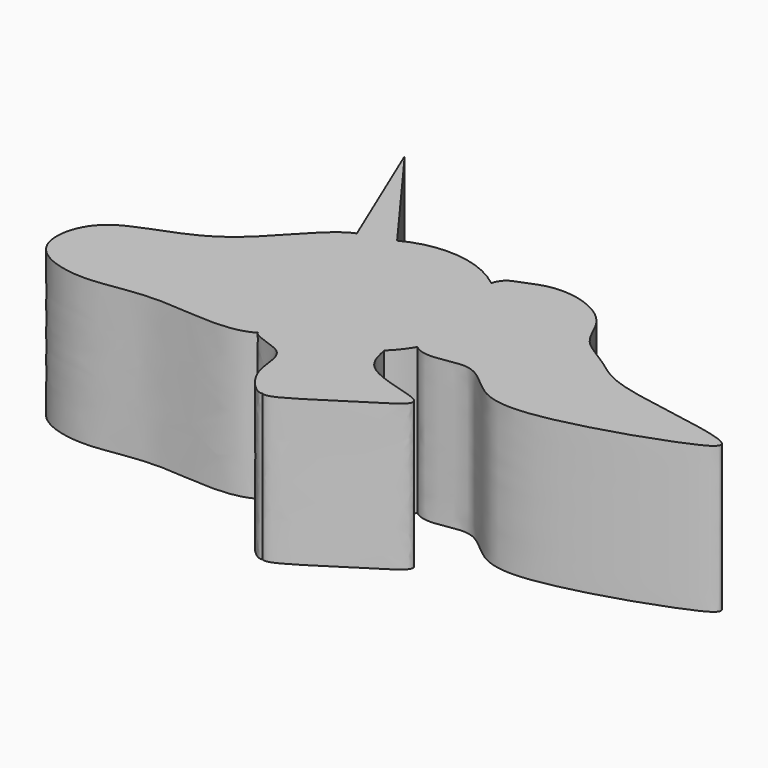
from build123d import *

# Parameters (mm, degrees)
F1_DEPTH = 25.4


with BuildPart() as f1:
    # F0 (on Top) → F1 (new body)
    with BuildSketch(Plane.XY):
        with BuildLine():
            ThreePointArc((15.6247597688, -17.5122784292), (16.158858904, -15.1511123847), (16.3382044071, -12.7369454131))
            ThreePointArc((16.3382044071, -12.7369454131), (14.732957367, -5.6745881247), (10.2326509171, 0))
            add(Edge.make_bspline(
                [(11.0694508842, -15.1028212661), (9.5993425881, -9.8895547332), (9.3093062782, -2.986619819), (10.2326509171, 0)],
                knots=[0.9266033138, 0.9266033138, 0.9266033138, 0.9266033138, 1, 1, 1, 1], degree=3))
            ThreePointArc((11.0694508842, -15.1028212661), (13.2014186834, -16.5829843604), (15.6247597688, -17.5122784292))
        make_face()
        with BuildLine():
            ThreePointArc((10.2326509171, 0), (14.732957367, -5.6745881247), (16.3382044071, -12.7369454131))
            ThreePointArc((16.3382044071, -12.7369454131), (16.158858904, -15.1511123847), (15.6247597688, -17.5122784292))
            ThreePointArc((15.6247597688, -17.5122784292), (24.9039357291, -15.5507675945), (29.064724865, -7.0279473439))
            ThreePointArc((29.064724865, -7.0279473439), (22.2178667073, 3.0289081499), (10.3511869131, 0.3453061453))
            add(Edge.make_bspline(
                [(10.2326509171, 0), (10.2701911189, 0.1214262863), (10.3097370055, 0.2363790128), (10.3511869131, 0.3453061453)],
                knots=[0, 0, 0, 0, 0.0029840715, 0.0029840715, 0.0029840715, 0.0029840715], degree=3))
        make_face()
        with BuildLine():
            add(Edge.make_bspline(
                [(11.0694508842, -15.1028212661), (9.5993425881, -9.8895547332), (9.3093062782, -2.986619819), (10.2326509171, 0)],
                knots=[0.9266033138, 0.9266033138, 0.9266033138, 0.9266033138, 1, 1, 1, 1], degree=3))
            ThreePointArc((10.2326509171, 0), (10.1764969932, 0.0449101719), (10.1201459651, 0.0895727775))
            ThreePointArc((10.1201459651, 0.0895727775), (7.4671185374, -7.7020590055), (11.0694508842, -15.1028212661))
        make_face()
        with BuildLine():
            ThreePointArc((29.064724865, -7.0279473439), (24.9039357291, -15.5507675945), (15.6247597688, -17.5122784292))
            ThreePointArc((15.6247597688, -17.5122784292), (14.97657106, -19.2668185001), (14.1320946898, -20.9357759959))
            add(Edge.make_bspline(
                [(10.3511869131, 0.3453061453), (10.9660918821, 1.9612285661), (13.1810710321, 2.5821615076), (17.4062250817, 4.5972614145), (23.5541211341, 4.0157306024), (29.1807841604, 0.4734658783), (30.6152690832, -5.6031749227), (37.2457146084, -8.7606918958), (41.6262591245, -13.5919512406), (69.4069767494, -16.0194865708), (58.4173073455, -21.3590816503), (43.2741615609, -26.3017495114), (29.7906561882, -27.9538614081), (23.9099000961, -18.8038777974), (16.6936052342, -23.0245011534), (14.1320946898, -20.9357759959)],
                knots=[0.0029840715, 0.0029840715, 0.0029840715, 0.0029840715, 0.0472524544, 0.0978197845, 0.156226181, 0.2156699733, 0.2729250454, 0.3328538195, 0.399296056, 0.5093923331, 0.5642444856, 0.6651313762, 0.7494833831, 0.8187715875, 0.8901220386, 0.8901220386, 0.8901220386, 0.8901220386], degree=3))
            ThreePointArc((10.3511869131, 0.3453061453), (22.2178667073, 3.0289081499), (29.064724865, -7.0279473439))
        make_face()
        with BuildLine():
            ThreePointArc((14.1320946898, -20.9357759959), (14.97657106, -19.2668185001), (15.6247597688, -17.5122784292))
            ThreePointArc((15.6247597688, -17.5122784292), (13.2014186834, -16.5829843604), (11.0694508842, -15.1028212661))
            add(Edge.make_bspline(
                [(14.1320946898, -20.9357759959), (12.8224019033, -19.8678169833), (11.8001572435, -17.6940364971), (11.0694508842, -15.1028212661)],
                knots=[0.8901220386, 0.8901220386, 0.8901220386, 0.8901220386, 0.9266033138, 0.9266033138, 0.9266033138, 0.9266033138], degree=3))
        make_face()
        with BuildLine():
            ThreePointArc((11.0694508842, -15.1028212661), (7.4671185374, -7.7020590055), (10.1201459651, 0.0895727775))
            ThreePointArc((10.1201459651, 0.0895727775), (1.5397794917, 3.5285395894), (-7.5334858124, 1.7607618112))
            ThreePointArc((-7.5334858124, 1.7607618112), (-8.9265880443, 0.947094529), (-10.2326509171, 0))
            add(Edge.make_bspline(
                [(-3.0699548582, -28.7841352111), (0.8240097012, -21.7530635718), (-4.4613062913, -2.497334585), (-10.2326509171, 0)],
                knots=[0.8075795969, 0.8075795969, 0.8075795969, 0.8075795969, 1, 1, 1, 1], degree=3))
            add(Edge.make_bspline(
                [(-1.0373402516, -29.0421853208), (-1.7263886536, -28.7488598338), (-2.411144298, -28.652496149), (-3.0699548582, -28.7841352111)],
                knots=[0.8274826523, 0.8274826523, 0.8274826523, 0.8274826523, 0.8828352089, 0.8828352089, 0.8828352089, 0.8828352089], degree=3))
            ThreePointArc((-1.0373402516, -29.0421853208), (0.2330522052, -29.0734875783), (1.5020347762, -29.0059593591))
            add(Edge.make_bspline(
                [(1.9966859836, -25.2967402339), (1.3467949947, -26.4147374297), (1.2639465735, -27.7023037912), (1.5020347762, -29.0059593591)],
                knots=[0, 0, 0, 0, 0.0539789023, 0.0539789023, 0.0539789023, 0.0539789023], degree=3))
            add(Edge.make_bspline(
                [(11.2626201962, -24.5729206396), (11.0063895855, -23.5189771031), (9.9645541492, -20.328136721), (3.5168312901, -22.6816582912), (1.9966859836, -25.2967402339)],
                knots=[0.8238879416, 0.8238879416, 0.8238879416, 0.8238879416, 0.873739171, 1, 1, 1, 1], degree=3))
            ThreePointArc((11.2626201962, -24.5729206396), (12.8269283667, -22.8565714892), (14.1320946898, -20.9357759959))
            add(Edge.make_bspline(
                [(14.1320946898, -20.9357759959), (12.8224019033, -19.8678169833), (11.8001572435, -17.6940364971), (11.0694508842, -15.1028212661)],
                knots=[0.8901220386, 0.8901220386, 0.8901220386, 0.8901220386, 0.9266033138, 0.9266033138, 0.9266033138, 0.9266033138], degree=3))
        make_face()
        with BuildLine():
            ThreePointArc((-10.2326509171, 0), (-8.9265880443, 0.947094529), (-7.5334858124, 1.7607618112))
            Line((-7.5334858124, 1.7607618112), (-22.2487710416, 21.8024943024))
            Line((-22.2487710416, 21.8024943024), (-13.127635327, 0))
            add(Edge.make_bspline(
                [(-10.2326509171, 0), (-11.1825010918, 0.4110123109), (-12.1455161813, 0.368094916), (-13.127635327, 0)],
                knots=[0, 0, 0, 0, 0.0316686258, 0.0316686258, 0.0316686258, 0.0316686258], degree=3))
        make_face()
        with BuildLine():
            add(Edge.make_bspline(
                [(6.2752948143, -44.7073355317), (7.4566317865, -45.6619770197), (16.6946003339, -38.7648248858), (28.6623877442, -32.6401294165), (12.4889474561, -31.4488202018), (11.6144968935, -26.0202815526), (11.2626201962, -24.5729206396)],
                knots=[0.3326677956, 0.3326677956, 0.3326677956, 0.3326677956, 0.483522904, 0.6092698166, 0.7554281822, 0.8238879416, 0.8238879416, 0.8238879416, 0.8238879416], degree=3))
            ThreePointArc((11.2626201962, -24.5729206396), (6.756260964, -27.6127600473), (1.5020347762, -29.0059593591))
            add(Edge.make_bspline(
                [(1.5020347762, -29.0059593591), (1.7582976885, -30.409130826), (2.3863654431, -31.8309416267), (3.0793600463, -33.0800123041)],
                knots=[0.0539789023, 0.0539789023, 0.0539789023, 0.0539789023, 0.1120783401, 0.1120783401, 0.1120783401, 0.1120783401], degree=3))
            add(Edge.make_bspline(
                [(3.7081294957, -34.1456867388), (3.5040593333, -33.7751099484), (3.2941622239, -33.4194445981), (3.0793600283, -33.0800122747)],
                knots=[0.6943378528, 0.6943378528, 0.6943378528, 0.6943378528, 0.7136660465, 0.7136660465, 0.7136660465, 0.7136660465], degree=3))
            add(Edge.make_bspline(
                [(3.7081294937, -34.1456867399), (4.9882228558, -36.1974885553), (6.3669138471, -37.6924416259), (6.2780647625, -40.2375798495), (6.2515850068, -40.5877476318)],
                knots=[0.1293935148, 0.1293935148, 0.1293935148, 0.1293935148, 0.2349709338, 0.2514569097, 0.2514569097, 0.2514569097, 0.2514569097], degree=3))
            add(Edge.make_bspline(
                [(6.2752948143, -44.7073355317), (6.8854909927, -44.3655439077), (6.7882111753, -42.687560365), (6.2515850082, -40.5877476332)],
                knots=[0.482945294, 0.482945294, 0.482945294, 0.482945294, 0.590468255, 0.590468255, 0.590468255, 0.590468255], degree=3))
        make_face()
        with BuildLine():
            ThreePointArc((1.5020347762, -29.0059593591), (6.756260964, -27.6127600473), (11.2626201962, -24.5729206396))
            add(Edge.make_bspline(
                [(11.2626201962, -24.5729206396), (11.0063895855, -23.5189771031), (9.9645541492, -20.328136721), (3.5168312901, -22.6816582912), (1.9966859836, -25.2967402339)],
                knots=[0.8238879416, 0.8238879416, 0.8238879416, 0.8238879416, 0.873739171, 1, 1, 1, 1], degree=3))
            add(Edge.make_bspline(
                [(1.9966859836, -25.2967402339), (1.3467949947, -26.4147374297), (1.2639465735, -27.7023037912), (1.5020347762, -29.0059593591)],
                knots=[0, 0, 0, 0, 0.0539789023, 0.0539789023, 0.0539789023, 0.0539789023], degree=3))
        make_face()
        with BuildLine():
            add(Edge.make_bspline(
                [(-3.0699548582, -28.7841352111), (0.8240097012, -21.7530635718), (-4.4613062913, -2.497334585), (-10.2326509171, 0)],
                knots=[0.8075795969, 0.8075795969, 0.8075795969, 0.8075795969, 1, 1, 1, 1], degree=3))
            ThreePointArc((-10.2326509171, 0), (-14.5067813584, -5.2209479499), (-16.3067587039, -11.7237604245))
            ThreePointArc((-16.3067587039, -11.7237604245), (-9.7227081214, -13.4309985411), (-6.8315372381, -19.5877440274))
            ThreePointArc((-6.8315372381, -19.5877440274), (-7.6120209178, -23.0344974741), (-9.8012018612, -25.808799349))
            ThreePointArc((-9.8012018612, -25.808799349), (-6.6052876316, -27.6804088185), (-3.0699548582, -28.7841352111))
        make_face()
        with BuildLine():
            ThreePointArc((-16.3067587039, -11.7237604245), (-14.5067813584, -5.2209479499), (-10.2326509171, 0))
            add(Edge.make_bspline(
                [(-10.2326509171, 0), (-11.1825010918, 0.4110123109), (-12.1455161813, 0.368094916), (-13.127635327, 0)],
                knots=[0, 0, 0, 0, 0.0316686258, 0.0316686258, 0.0316686258, 0.0316686258], degree=3))
            add(Edge.make_bspline(
                [(-13.127635327, 0), (-16.9885407298, -1.4470542155), (-26.1475214336, -15.710526233), (-43.4116839601, -16.662992314), (-45.950942929, -30.8867076179), (-33.5443465173, -34.5459712582), (-23.2656635988, -30.7793989739), (-9.4186082957, -33.630807497), (-5.3864327744, -31.188833942)],
                knots=[0.0316686258, 0.0316686258, 0.0316686258, 0.0316686258, 0.1561642831, 0.3060221782, 0.4153421079, 0.5268671977, 0.655086979, 0.7787124677, 0.7787124677, 0.7787124677, 0.7787124677], degree=3))
            add(Edge.make_bspline(
                [(-3.0699548582, -28.7841352111), (-4.4644595819, -29.062775696), (-5.7427193917, -30.362964597), (-5.3864327744, -31.188833942)],
                knots=[0.8828352089, 0.8828352089, 0.8828352089, 0.8828352089, 1, 1, 1, 1], degree=3))
            ThreePointArc((-3.0699548582, -28.7841352111), (-6.6052876316, -27.6804088185), (-9.8012018612, -25.808799349))
            ThreePointArc((-9.8012018612, -25.808799349), (-22.0961404136, -22.9426465286), (-16.3067587039, -11.7237604245))
        make_face()
        with BuildLine():
            add(Edge.make_bspline(
                [(1.5020347762, -29.0059593591), (1.7582976885, -30.409130826), (2.3863654431, -31.8309416267), (3.0793600463, -33.0800123041)],
                knots=[0.0539789023, 0.0539789023, 0.0539789023, 0.0539789023, 0.1120783401, 0.1120783401, 0.1120783401, 0.1120783401], degree=3))
            ThreePointArc((1.5020347762, -29.0059593591), (0.2330522052, -29.0734875783), (-1.0373402516, -29.0421853208))
            add(Edge.make_bspline(
                [(3.0793600463, -33.0800123041), (1.8144691163, -31.0812204976), (0.3794895238, -29.6453247849), (-1.0373402516, -29.0421853208)],
                knots=[0.7136660465, 0.7136660465, 0.7136660465, 0.7136660465, 0.8274826523, 0.8274826523, 0.8274826523, 0.8274826523], degree=3))
        make_face()
        with BuildLine():
            add(Edge.make_bspline(
                [(-5.3864327744, -31.188833942), (-4.908330002, -32.2970720971), (2.1683533748, -32.8226904652), (0.3871749857, -40.3054793101), (5.3800366063, -45.2088000896), (6.2752948143, -44.7073355317)],
                knots=[0, 0, 0, 0, 0.1572240121, 0.3251914161, 0.482945294, 0.482945294, 0.482945294, 0.482945294], degree=3))
            add(Edge.make_bspline(
                [(6.2515850082, -40.5877476332), (6.1211441743, -42.3126947019), (5.6393374171, -44.1934167006), (6.2752948143, -44.7073355317)],
                knots=[0.2514569097, 0.2514569097, 0.2514569097, 0.2514569097, 0.3326677956, 0.3326677956, 0.3326677956, 0.3326677956], degree=3))
            add(Edge.make_bspline(
                [(6.2515850082, -40.5877476332), (5.7331920658, -38.5592813245), (4.8048013486, -36.1371642314), (3.7081294957, -34.1456867388)],
                knots=[0.590468255, 0.590468255, 0.590468255, 0.590468255, 0.6943378528, 0.6943378528, 0.6943378528, 0.6943378528], degree=3))
            add(Edge.make_bspline(
                [(3.0793600463, -33.0800123041), (3.2858908332, -33.4522685219), (3.4981884, -33.8091819739), (3.7081294937, -34.1456867399)],
                knots=[0.1120783401, 0.1120783401, 0.1120783401, 0.1120783401, 0.1293935148, 0.1293935148, 0.1293935148, 0.1293935148], degree=3))
            add(Edge.make_bspline(
                [(3.0793600463, -33.0800123041), (1.8144691163, -31.0812204976), (0.3794895238, -29.6453247849), (-1.0373402516, -29.0421853208)],
                knots=[0.7136660465, 0.7136660465, 0.7136660465, 0.7136660465, 0.8274826523, 0.8274826523, 0.8274826523, 0.8274826523], degree=3))
            ThreePointArc((-1.0373402516, -29.0421853208), (-2.0576967086, -28.9450547261), (-3.0699548582, -28.7841352111))
            add(Edge.make_bspline(
                [(-5.3864327744, -31.188833942), (-4.4449009501, -30.618621707), (-3.6541318811, -29.838944631), (-3.0699548582, -28.7841352111)],
                knots=[0.7787124677, 0.7787124677, 0.7787124677, 0.7787124677, 0.8075795969, 0.8075795969, 0.8075795969, 0.8075795969], degree=3))
        make_face()
        with BuildLine():
            add(Edge.make_bspline(
                [(6.2515850082, -40.5877476332), (6.1211441743, -42.3126947019), (5.6393374171, -44.1934167006), (6.2752948143, -44.7073355317)],
                knots=[0.2514569097, 0.2514569097, 0.2514569097, 0.2514569097, 0.3326677956, 0.3326677956, 0.3326677956, 0.3326677956], degree=3))
            add(Edge.make_bspline(
                [(6.2752948143, -44.7073355317), (6.8854909927, -44.3655439077), (6.7882111753, -42.687560365), (6.2515850082, -40.5877476332)],
                knots=[0.482945294, 0.482945294, 0.482945294, 0.482945294, 0.590468255, 0.590468255, 0.590468255, 0.590468255], degree=3))
        make_face()
        with BuildLine():
            ThreePointArc((-6.8315372381, -19.5877440274), (-9.7227081214, -13.4309985411), (-16.3067587039, -11.7237604245))
            ThreePointArc((-16.3067587039, -11.7237604245), (-14.8325143382, -19.5877440274), (-9.8012018612, -25.808799349))
            ThreePointArc((-9.8012018612, -25.808799349), (-7.6120209178, -23.0344974741), (-6.8315372381, -19.5877440274))
        make_face()
        with BuildLine():
            ThreePointArc((-9.8012018612, -25.808799349), (-14.8325143382, -19.5877440274), (-16.3067587039, -11.7237604245))
            ThreePointArc((-16.3067587039, -11.7237604245), (-22.0961404136, -22.9426465286), (-9.8012018612, -25.808799349))
        make_face()
        with BuildLine():
            add(Edge.make_bspline(
                [(-1.0373402516, -29.0421853208), (-1.7263886536, -28.7488598338), (-2.411144298, -28.652496149), (-3.0699548582, -28.7841352111)],
                knots=[0.8274826523, 0.8274826523, 0.8274826523, 0.8274826523, 0.8828352089, 0.8828352089, 0.8828352089, 0.8828352089], degree=3))
            ThreePointArc((-3.0699548582, -28.7841352111), (-2.0576967086, -28.9450547261), (-1.0373402516, -29.0421853208))
        make_face()
        with BuildLine():
            add(Edge.make_bspline(
                [(-5.3864327744, -31.188833942), (-4.4449009501, -30.618621707), (-3.6541318811, -29.838944631), (-3.0699548582, -28.7841352111)],
                knots=[0.7787124677, 0.7787124677, 0.7787124677, 0.7787124677, 0.8075795969, 0.8075795969, 0.8075795969, 0.8075795969], degree=3))
            add(Edge.make_bspline(
                [(-3.0699548582, -28.7841352111), (-4.4644595819, -29.062775696), (-5.7427193917, -30.362964597), (-5.3864327744, -31.188833942)],
                knots=[0.8828352089, 0.8828352089, 0.8828352089, 0.8828352089, 1, 1, 1, 1], degree=3))
        make_face()
        with BuildLine():
            add(Edge.make_bspline(
                [(6.2515850082, -40.5877476332), (5.7331920658, -38.5592813245), (4.8048013486, -36.1371642314), (3.7081294957, -34.1456867388)],
                knots=[0.590468255, 0.590468255, 0.590468255, 0.590468255, 0.6943378528, 0.6943378528, 0.6943378528, 0.6943378528], degree=3))
            add(Edge.make_bspline(
                [(3.7081294937, -34.1456867399), (4.9882228558, -36.1974885553), (6.3669138471, -37.6924416259), (6.2780647625, -40.2375798495), (6.2515850068, -40.5877476318)],
                knots=[0.1293935148, 0.1293935148, 0.1293935148, 0.1293935148, 0.2349709338, 0.2514569097, 0.2514569097, 0.2514569097, 0.2514569097], degree=3))
        make_face()
    extrude(amount=F1_DEPTH)


solid = f1.part
